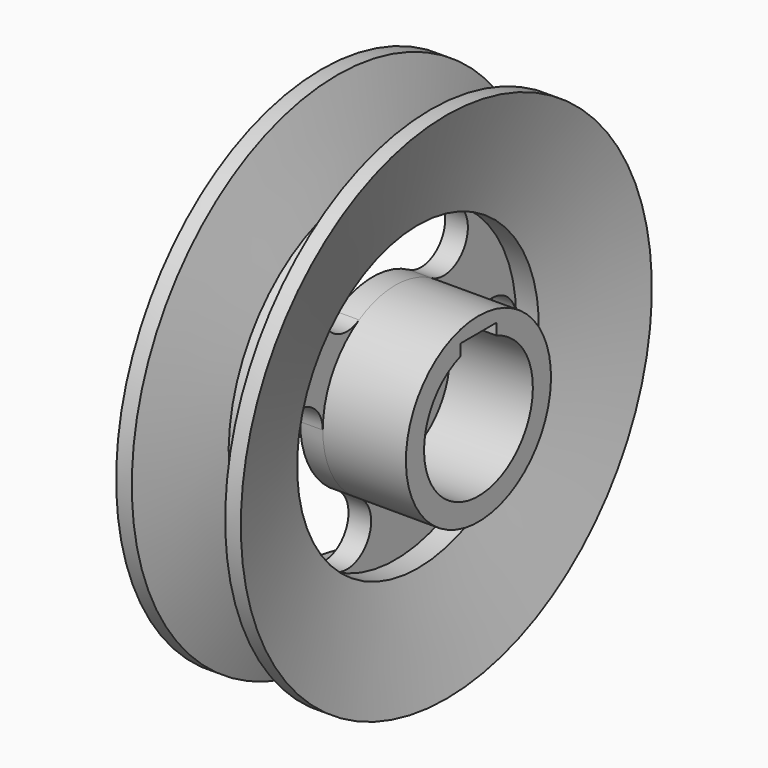
from build123d import *

# Parameters (mm, degrees)
F2_W     = 6
F2_H     = 2
F3_DEPTH = 11
F5_DEPTH = 25


# Not quite as in the source:
# - after a boolean that leaves OpenCascade's solid faulty, fix() repairs it


with BuildPart() as f1:
    # F0 (on Front) → F1 (revolve)
    with BuildSketch(Plane.XZ):
        Polygon((8.25, 34), (6.179448, 34), (2.964057, 22), (0, 22), (-2.964057, 22), (-6.179448, 34), (-8.25, 34), (-4.498711, 20), (-1.5, 20), (-1.5, 4), (1.5, 4), (1.5, 9), (12.5, 9), (12.5, 12), (1.5, 12), (1.5, 20), (4.498711, 20), align=None)
    revolve(axis=Axis((3.581624, 0, 0), (1, 0, 0)))

    # F2 (on face) → F3 (cut)
    with BuildSketch(Plane.YZ.offset(12.5)):
        with Locations((0, 9)):
            Rectangle(F2_W, F2_H)
    extrude(amount=-F3_DEPTH, mode=Mode.SUBTRACT)

    # F4 (on face) → F5 (cut)
    with BuildSketch(Plane.YZ.offset(1.5)):
        with BuildLine():
            ThreePointArc((-12, 0), (-16, 4), (-20, 0))
            ThreePointArc((-20, 0), (-17.320508, -10), (-10, -17.320508))
            ThreePointArc((-10, -17.320508), (-4.535898, -15.856406), (-6, -10.392305))
            ThreePointArc((-6, -10.392305), (-10.392305, -6), (-12, 0))
        make_face()
        with BuildLine():
            ThreePointArc((10, 17.320508), (0, 20), (-10, 17.320508))
            ThreePointArc((-10, 17.320508), (-11.464102, 11.856406), (-6, 10.392305))
            ThreePointArc((-6, 10.392305), (0, 12), (6, 10.392305))
            ThreePointArc((6, 10.392305), (11.464102, 11.856406), (10, 17.320508))
        make_face()
        with BuildLine():
            ThreePointArc((6, -10.392305), (4.535898, -15.856406), (10, -17.320508))
            ThreePointArc((10, -17.320508), (17.320508, -10), (20, 0))
            ThreePointArc((20, 0), (16, 4), (12, 0))
            ThreePointArc((12, 0), (10.392305, -6), (6, -10.392305))
        make_face()
    extrude(amount=-F5_DEPTH, mode=Mode.SUBTRACT)

    add(f1.part.fix(), mode=Mode.REPLACE)


solid = f1.part
